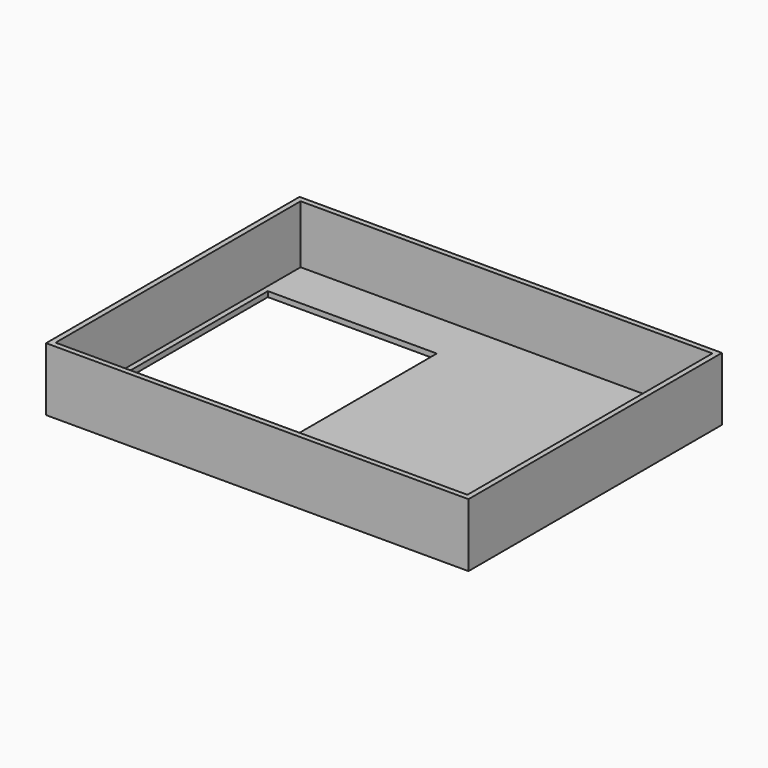
from build123d import *

# Parameters (mm, degrees)
F0_W     = 508
F0_H     = 381
F1_DEPTH = 76.2
F2_W     = 203.2
F2_H     = 254
F3_DEPTH = 76.2
F4_T     = -6.35
F5_W     = 215.9
F5_H     = 266.7
F5_W_2   = 203.2
F5_H_2   = 254
F6_DEPTH = 69.85


# Not quite as in the source:
# - a shell that OpenCascade refuses in one call is made with other operations: the cavity is built on its own and cut out


with BuildPart() as f1:
    # F0 (on Top) → F1 (new body)
    with BuildSketch(Plane.XY):
        Rectangle(F0_W, F0_H)
    extrude(amount=F1_DEPTH)

    # F2 (on face) → F3 (cut, through all)
    with BuildSketch(Plane.XY.offset(76.2)):
        with Locations((-139.7, 0)):
            Rectangle(F2_W, F2_H)
    extrude(amount=-F3_DEPTH, mode=Mode.SUBTRACT)

    # F4: a shell. OpenCascade refuses it in one call, so the cavity is built on its own and cut out:
    # the body offset inwards by the wall thickness, plus a prism from it out through each open face.
    f4_core = offset(f1.part, amount=F4_T, kind=Kind.INTERSECTION, mode=Mode.PRIVATE)
    f4_exits = [f4_core.faces().sort_by_distance(p)[0] for p in [
        (64.435271, 0, 69.85),
    ]]
    add(f4_core, mode=Mode.SUBTRACT)
    extrude(f4_exits, amount=-F4_T, mode=Mode.SUBTRACT)

    # F5 (on face) → F6 (cut)
    with BuildSketch(Plane.XY.offset(76.2)):
        with Locations((-139.7, 0)):
            Rectangle(F5_W, F5_H)
        with Locations((-139.7, 0)):
            Rectangle(F5_W_2, F5_H_2, mode=Mode.SUBTRACT)
    extrude(amount=-F6_DEPTH, mode=Mode.SUBTRACT)


solid = f1.part
